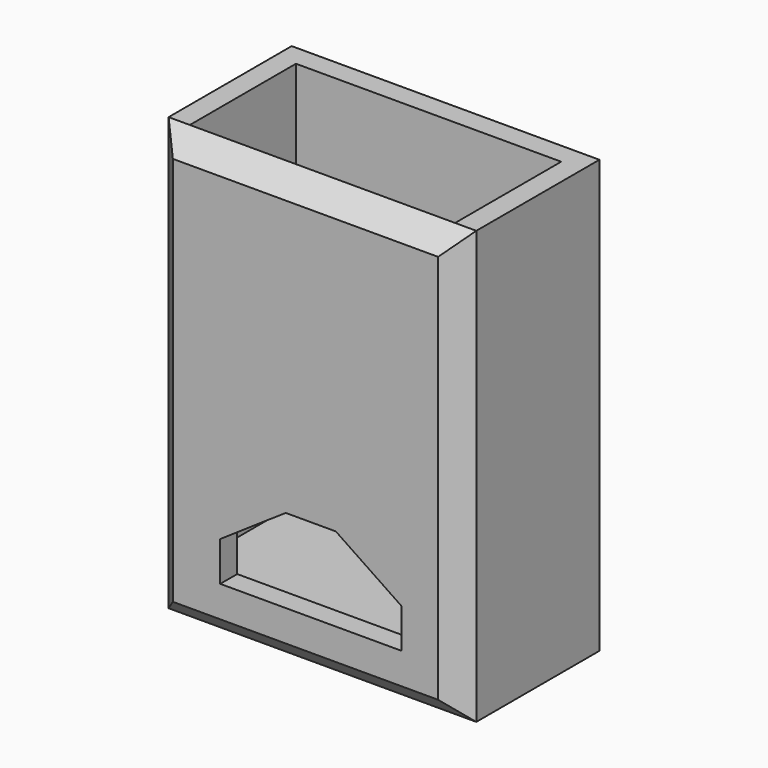
from build123d import *

# Parameters (mm, degrees)
F0_W     = 29
F0_H     = 16.5
F1_DEPTH = 38.5
F2_T     = -2
F3_DEPTH = 2.25
F4_SIZE  = 1.99999
F6_DEPTH = 25


# Not quite as in the source:
# - a fillet or chamfer is up to 0.001 mm smaller than in the source, because OpenCascade refuses the exact size


with BuildPart() as f1:
    # F0 (on Top) → F1 (new body)
    with BuildSketch(Plane.XY):
        with Locations((14.5, 8.25)):
            Rectangle(F0_W, F0_H)
    extrude(amount=F1_DEPTH)

    # F2
    f2_openings = [f1.faces().sort_by_distance(p)[0] for p in [
        (14.5, 8.25, 38.5),
    ]]
    offset(amount=F2_T, openings=f2_openings)

    # F3 (add): a face of the model
    f3_faces = [f1.faces().sort_by_distance(p)[0] for p in [
        (14.5, 8.25, 0),
    ]]
    extrude(f3_faces, amount=F3_DEPTH)

    # F4 (size 2 in the source; OpenCascade refuses exactly that, so slightly less here)
    f4_edges = [f1.edges().sort_by_distance(p)[0] for p in [
        (29, 0, 18.125),
        (0, 0, 18.125),
        (14.5, 0, 38.5),
        (14.5, 0, -2.25),
    ]]
    chamfer(f4_edges, length=F4_SIZE)

    # F5 (on face) → F6 (cut)
    with BuildSketch(Plane.XZ):
        Polygon((17.364, 10.584), (12.635, 10.584), (6.464, 6.414), (6.464, 2.69), (23.536, 2.69), (23.536, 6.414), align=None)
    extrude(amount=-F6_DEPTH, mode=Mode.SUBTRACT)


solid = f1.part
